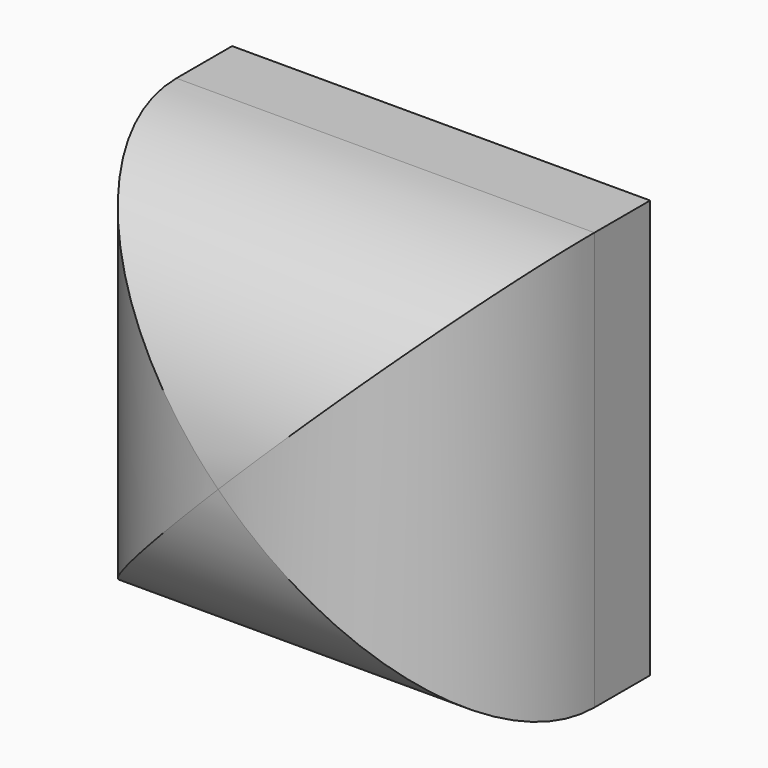
from build123d import *

# Parameters (mm, degrees)
F0_W     = 30
F0_H     = 30
F1_DEPTH = 20
F2_R     = 14.99999


# Not quite as in the source:
# - a fillet or chamfer is up to 0.001 mm smaller than in the source, because OpenCascade refuses the exact size


with BuildPart() as f1:
    # F0 (on Front) → F1 (new body)
    with BuildSketch(Plane.XZ):
        with Locations((0.0142654032, 1.3629881293)):
            Rectangle(F0_W, F0_H)
    extrude(amount=F1_DEPTH)

    # F2 (radius 15 in the source; OpenCascade refuses exactly that, so slightly less here)
    f2_edges = [f1.edges().sort_by_distance(p)[0] for p in [
        (0.014265, -20, -13.637012),
        (15.014265, -20, 1.362988),
        (0.014265, -20, 16.362988),
        (-14.985735, -20, 1.362988),
    ]]
    fillet(f2_edges, radius=F2_R)


solid = f1.part
